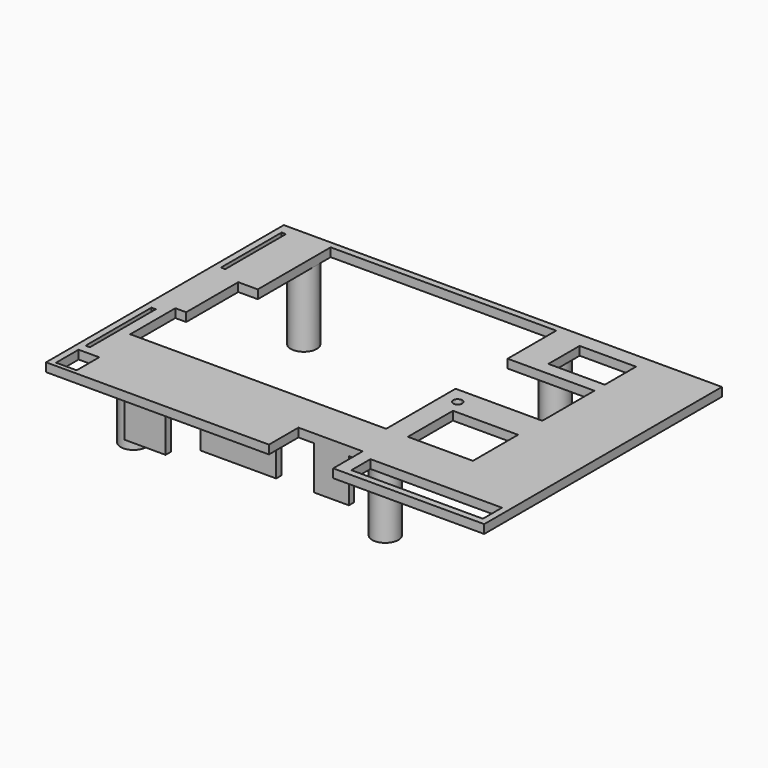
from build123d import *

# Parameters (mm, degrees)
F0_W      = 89
F0_H      = 60
F1_DEPTH  = 2
F2_R      = 3
F2_R_2    = 1.5
F3_DEPTH  = 17
F4_W      = 52
F4_H      = 49
F5_DEPTH  = 2
F6_W      = 4.5
F6_H      = 15
F7_DEPTH  = 2
F8_W      = 14.81
F8_H      = 10
F9_DEPTH  = 2
F11_W     = 17.5
F11_H     = 1.5
F11_W_2   = 8
F12_DEPTH = 10
F11_W_3   = 9.5
F13_DEPTH = 13.5
F14_W     = 1.5
F14_H     = 4
F15_DEPTH = 4
F16_SIZE  = 3.99999
F17_W     = 20
F17_H     = 15
F18_DEPTH = 2
F19_W     = 15
F19_H     = 13
F19_W_2   = 30.315
F19_H_2   = 5.5
F19_W_3   = 13
F19_H_3   = 9
F20_DEPTH = 2
F22_W     = 4.75
F22_H     = 6.5
F22_W_2   = 1
F22_H_2   = 19
F22_H_3   = 17.5
F23_DEPTH = 2
F25_DEPTH = 2
F21_R     = 1.05
F26_DEPTH = 2


# Not quite as in the source:
# - a fillet or chamfer is up to 0.001 mm smaller than in the source, because OpenCascade refuses the exact size
# - a feature of the source that left no trace in its solid (it failed there, or was rolled back) is left out


with BuildPart() as f1:
    # F0 (on Top) → F1 (new body)
    with BuildSketch(Plane.XY):
        Polygon((89, 0), (0, 0), (0, 60), (-5, 60), (-5, 0), (-5, -10), (89, -10), (99, -10), (99, 60), (89, 60), align=None)
        Polygon((-5, 60), (0, 60), (89, 60), (99, 60), (99, 61.5), (-5, 61.5), align=None)
        with Locations((44.5, 30)):
            Rectangle(F0_W, F0_H)
    extrude(amount=F1_DEPTH)

    # F2 (on face) → F3 (join)
    with BuildSketch(Plane(origin=(0, 0, 0), x_dir=(1, 0, 0), z_dir=(0, 0, -1))):
        with Locations((5.5, -5.5)):
            Circle(F2_R)
        with Locations((5.5, -5.5)):
            Circle(F2_R_2, mode=Mode.SUBTRACT)
        with Locations((63.5, -5.5)):
            Circle(F2_R)
        with Locations((63.5, -5.5)):
            Circle(F2_R_2, mode=Mode.SUBTRACT)
        with Locations((5.5, -54.5)):
            Circle(F2_R)
        with Locations((5.5, -54.5)):
            Circle(F2_R_2, mode=Mode.SUBTRACT)
        with Locations((63.5, -54.5)):
            Circle(F2_R)
        with Locations((63.5, -54.5)):
            Circle(F2_R_2, mode=Mode.SUBTRACT)
    extrude(amount=F3_DEPTH)

    # F4 (on face) → F5 (cut, through all)
    with BuildSketch(Plane.XY.offset(2)):
        with Locations((34.5, 34)):
            Rectangle(F4_W, F4_H)
    extrude(amount=-F5_DEPTH, mode=Mode.SUBTRACT)

    # F6 (on face) → F7 (cut, through all)
    with BuildSketch(Plane.XY.offset(2)):
        with Locations((6.25, 30)):
            Rectangle(F6_W, F6_H)
        Polygon((8.5, 9.5), (8.5, 22.5), (4, 22.5), (1.5, 22.5), (1.5, 9.5), align=None)
    extrude(amount=-F7_DEPTH, mode=Mode.SUBTRACT)

    # F8 (on face) → F9 (cut, through all)
    with BuildSketch(Plane.XY.offset(2)):
        with Locations((55.28, -5)):
            Rectangle(F8_W, F8_H)
    extrude(amount=-F9_DEPTH, mode=Mode.SUBTRACT)

    # F11 (on face) → F12 (join)
    with BuildSketch(Plane(origin=(0, 0, 0), x_dir=(1, 0, 0), z_dir=(0, 0, -1))):
        with Locations((34, -0.75)):
            Rectangle(F11_W, F11_H)
        with Locations((55.5, -0.75)):
            Rectangle(F11_W_2, F11_H)
    extrude(amount=F12_DEPTH)

    # F11 (on face) → F13 (join)
    with BuildSketch(Plane(origin=(0, 0, 0), x_dir=(1, 0, 0), z_dir=(0, 0, -1))):
        with Locations((12.5, -0.75)):
            Rectangle(F11_W_3, F11_H)
    extrude(amount=F13_DEPTH)

    # F14 (on face) → F15 (join)
    with BuildSketch(Plane(origin=(0, 0, 0), x_dir=(1, 0, 0), z_dir=(0, 0, -1))):
        with Locations((34, -3.5)):
            Rectangle(F14_W, F14_H)
        with Locations((55.5, -3.5)):
            Rectangle(F14_W, F14_H)
        with Locations((12.5, -3.5)):
            Rectangle(F14_W, F14_H)
    extrude(amount=F15_DEPTH)

    # F16 (size 4 in the source; OpenCascade refuses exactly that, so slightly less here)
    f16_edges = [f1.edges().sort_by_distance(p)[0] for p in [
        (12.5, 5.5, -4),
        (34, 5.5, -4),
        (55.5, 5.5, -4),
    ]]
    chamfer(f16_edges, length=F16_SIZE)

    # F17 (on face) → F18 (cut, through all)
    with BuildSketch(Plane(origin=(0, 0, 0), x_dir=(1, 0, 0), z_dir=(0, 0, -1))):
        with Locations((70.5, -37)):
            Rectangle(F17_W, F17_H)
    extrude(amount=-F18_DEPTH, mode=Mode.SUBTRACT)

    # F19 (on face) → F20 (cut, through all)
    with BuildSketch(Plane(origin=(0, 0, 0), x_dir=(1, 0, 0), z_dir=(0, 0, -1))):
        with Locations((73, -16)):
            Rectangle(F19_W, F19_H)
        with Locations((80.8425, 4.25)):
            Rectangle(F19_W_2, F19_H_2)
        with Locations((74, -52)):
            Rectangle(F19_W_3, F19_H_3)
    extrude(amount=-F20_DEPTH, mode=Mode.SUBTRACT)

    # F22 (on face) → F23 (cut, through all)
    with BuildSketch(Plane.XY):
        with Locations((0.375, -4.25)):
            Rectangle(F22_W, F22_H)
        with Locations((-1.5, 10.5)):
            Rectangle(F22_W_2, F22_H_2)
        with Locations((-1.5, 48.75)):
            Rectangle(F22_W_2, F22_H_3)
    extrude(amount=F23_DEPTH, mode=Mode.SUBTRACT)

    # F24 (on face) → F25 (cut, through all)
    with BuildSketch(Plane.XY.offset(2)):
        Polygon((-3.5, -8.5), (-3.5, 60), (97.5, 60), (97.5, -8.5), (62.685, -8.5), (62.685, -10), (99, -10), (99, 61.5), (-5, 61.5), (-5, -10), (47.875, -10), (47.875, -8.5), align=None)
    extrude(amount=-F25_DEPTH, mode=Mode.SUBTRACT)

    # F21 (on face) → F26 (cut, through all)
    with BuildSketch(Plane.XY.offset(2)):
        with BuildLine():
            ThreePointArc((64, 24.7), (64.7424621202, 25.0075378798), (65.05, 25.75))
            ThreePointArc((65.05, 25.75), (64.7424621202, 26.4924621202), (64, 26.8))
            Line((64, 26.8), (64, 25.75))
            Line((64, 25.75), (64, 24.7))
        make_face()
        with BuildLine():
            Line((64, 25.75), (64, 26.8))
            ThreePointArc((64, 26.8), (62.95, 25.75), (64, 24.7))
            Line((64, 24.7), (64, 25.75))
        make_face()
        with Locations((44, 14.5)):
            Circle(F21_R)
    extrude(amount=-F26_DEPTH, mode=Mode.SUBTRACT)


solid = f1.part
